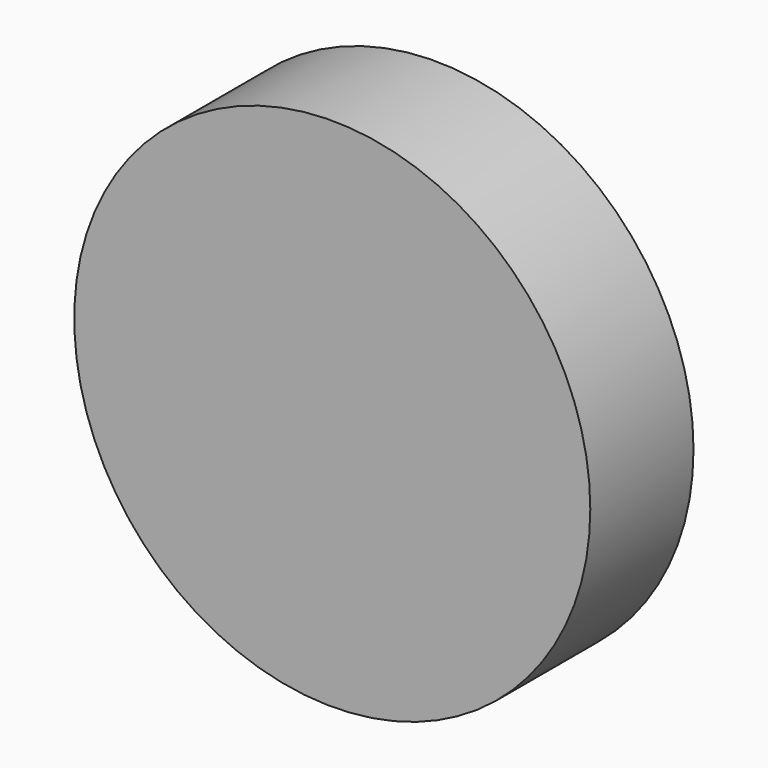
from build123d import *

# Parameters (mm, degrees)
F0_R     = 100
F1_DEPTH = 50


# Not quite as in the source:
# - a feature names something its author has since deleted; it is built from what else it names


with BuildPart() as f1:
    # F0 (on Front) → F1 (new body)
    with BuildSketch(Plane.XZ):
        Circle(F0_R)
    extrude(amount=F1_DEPTH)


solid = f1.part
